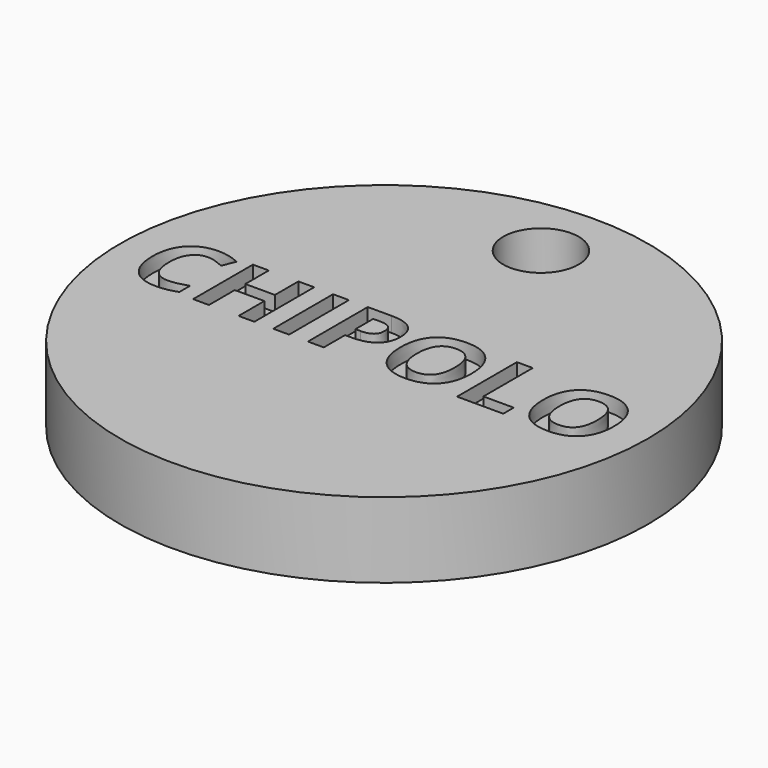
from build123d import *

# Parameters (mm, degrees)
F0_R         = 17.5
F1_DEPTH     = 5
F2_TEXT_SIZE = 6.9444444444
F3_DEPTH     = 1
F4_R         = 2.5
F5_DEPTH     = 25


# Not quite as in the source:
# - Text() gives the source's letters only with a copy of the font that has no kerning and outlines rounded to 1/6400 em; it was checked with that copy


with BuildPart() as f1:
    # F0 (on Top) → F1 (new body)
    with BuildSketch(Plane.XY):
        Circle(F0_R)
    extrude(amount=F1_DEPTH)

    # F2 (on face) → F3 (cut)
    with BuildSketch(Plane.XY.offset(5)):
        with Locations((-15.7118055556, -2.5)):
            Text('CHIPOLO', F2_TEXT_SIZE, font='Open Sans', font_style=FontStyle.BOLD, text_align=(TextAlign.LEFT, TextAlign.BOTTOM))
    extrude(amount=-F3_DEPTH, mode=Mode.SUBTRACT)

    # F4 (on face) → F5 (cut)
    with BuildSketch(Plane.XY.offset(5)):
        with Locations((0, 13)):
            Circle(F4_R)
    extrude(amount=-F5_DEPTH, mode=Mode.SUBTRACT)


solid = f1.part
